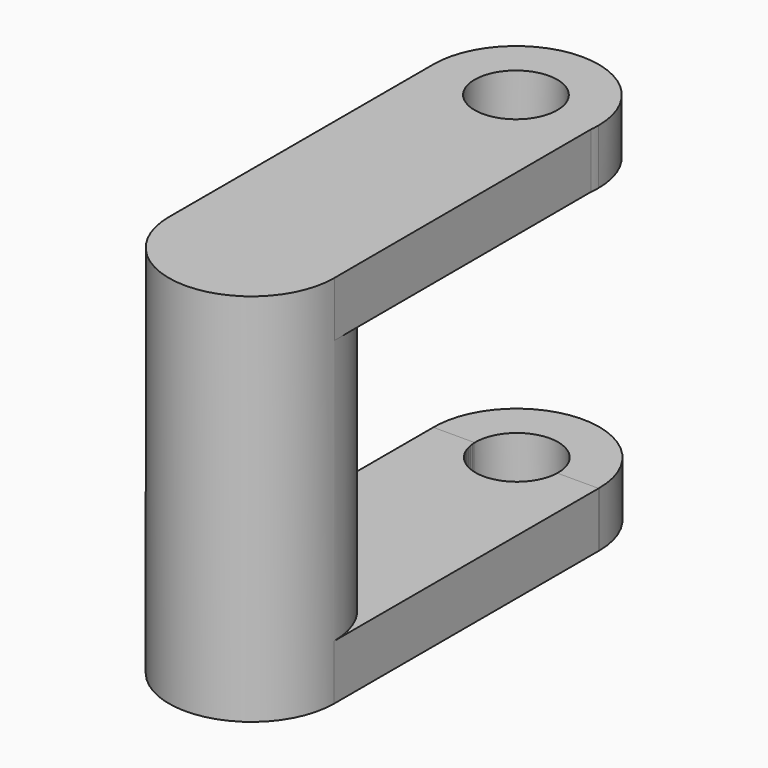
from build123d import *

# Parameters (mm, degrees)
F0_R     = 76.2
F4_DEPTH = 345.44
F6_DEPTH = 50.8
F7_DEPTH = 50.8
F3_R     = 38.1
F8_DEPTH = 91.44


# Not quite as in the source:
# - ends of sketch curves that miss each other by under 0.0002 mm in the source are joined


with BuildPart() as f4:
    # F0 (on Top) → F4 (new body)
    with BuildSketch(Plane.XY):
        Circle(F0_R)
    extrude(amount=F4_DEPTH)

    # F5 (on face) → F6 (join)
    with BuildSketch(Plane.XY.offset(345.44)):
        with BuildLine():
            ThreePointArc((-76.2, 304.8), (-4.2065849822, 228.7161998663), (75.7355549288, 296.399659553))
            Line((75.7355549288, 296.399659553), (75.7223893169, 304.8))
            Line((75.7223893169, 304.8), (38.1, 304.8))
            ThreePointArc((38.1, 304.8), (0, 266.7), (-38.1, 304.8))
            Line((-38.1, 304.8), (-76.2, 304.8))
        make_face()
        with BuildLine():
            Line((75.7223893169, 304.8), (75.7355549288, 296.399659553))
            ThreePointArc((75.7355549288, 296.399659553), (76.0838001337, 300.5934150178), (76.2, 304.8))
            ThreePointArc((76.2, 304.8), (0, 381), (-76.2, 304.8))
            Line((-76.2, 304.8), (-38.1, 304.8))
            ThreePointArc((-38.1, 304.8), (0, 342.9), (38.1, 304.8))
            Line((38.1, 304.8), (75.7223893169, 304.8))
        make_face()
        with BuildLine():
            ThreePointArc((-76.2, 0), (0, 76.2), (76.2, 0))
            Line((76.2, 0), (75.7355549288, 296.399659553))
            ThreePointArc((75.7355549288, 296.399659553), (-4.2065849822, 228.7161998663), (-76.2, 304.8))
            Line((-76.2, 304.8), (-76.2, 0))
        make_face()
    extrude(amount=-F6_DEPTH)


with BuildPart() as f7:
    # F2 (on face) → F7 (new body)
    with BuildSketch(Plane.XY):
        with BuildLine():
            Line((-76.1898637822, 304.8), (-76.1898637822, 304.3581831019))
            ThreePointArc((-76.1898637822, 304.3581831019), (0.2209283182, 229.401345622), (76.1957896369, 304.8))
            Line((76.1957896369, 304.8), (-76.1898637822, 304.8))
        make_face()
        with BuildLine():
            ThreePointArc((76.1957896369, 304.8), (76.198947402, 305.2005071425), (76.2, 305.6010253502))
            ThreePointArc((76.2, 305.6010253502), (-0.6214417907, 381.7984912536), (-76.1898637822, 304.3581831019))
            Line((-76.1898637822, 304.3581831019), (-76.1898637822, 304.8))
            Line((-76.1898637822, 304.8), (76.1957896369, 304.8))
        make_face()
    extrude(amount=F7_DEPTH)


with BuildPart() as f7b:
    # F1 (on Top) → F7, piece 2 (new body)
    with BuildSketch(Plane.XY):
        Polygon((-76.1898637822, 0), (0, 0), (76.2101362178, 0), (76.2101362178, 304.8), (-76.1898637822, 304.8), align=None)
    extrude(amount=F7_DEPTH)


with BuildPart() as f8_tool:
    # F3 (on face) → F8 (new body)
    with BuildSketch(Plane.XY):
        with Locations((0, 305.761307478)):
            Circle(F3_R)
    extrude(amount=F8_DEPTH)


with BuildPart() as f7_1:
    add(f7.part)

    # F8: cut by f8_tool
    add(f8_tool.part, mode=Mode.SUBTRACT)


with BuildPart() as f7b_1:
    add(f7b.part)

    # F8: cut by f8_tool
    add(f8_tool.part, mode=Mode.SUBTRACT)


solid = Compound([f4.part, f7_1.part, f7b_1.part])
